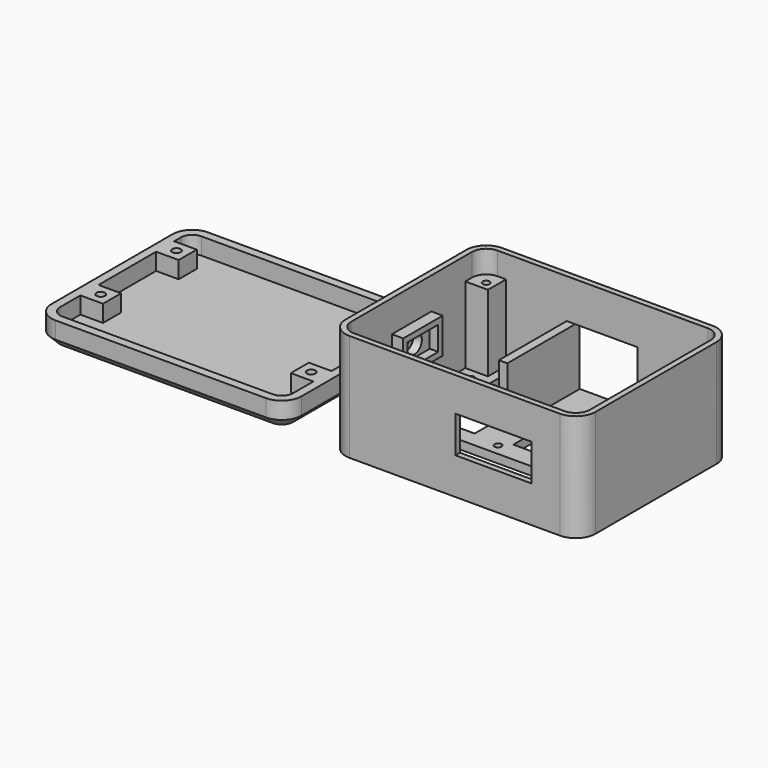
from build123d import *

# Parameters (mm, degrees)
F0_R      = 1.5
F1_DEPTH  = 3
F2_DEPTH  = 38
F0_R_2    = 1.25
F3_DEPTH  = 30
F4_W      = 21
F4_H      = 17
F5_DEPTH  = 7
F7_DEPTH  = 3
F8_W      = 4
F8_H      = 9
F9_DEPTH  = 25
F10_SIZE  = 1.5
F12_W     = 21
F12_H     = 21
F13_DEPTH = 25
F14_DEPTH = 25
F15_R     = 1.5
F15_R_2   = 1.25
F16_DEPTH = 3
F15_W     = 8
F15_H     = 8
F17_DEPTH = 9
F18_SIZE  = 3
F19_DEPTH = 25
F8_W_2    = 17.5
F8_H_2    = 12.5
F8_W_3    = 13.5
F8_H_3    = 8.5
F20_DEPTH = 4
F8_R      = 3.25
F21_DEPTH = 25
F23_DEPTH = 8
F24_DEPTH = 1
F25_DEPTH = 1
F26_DEPTH = 1
F27_DEPTH = 1
F28_DEPTH = 1
F29_W     = 3
F29_H     = 30
F30_DEPTH = 21
F31_DEPTH = 1
F29_W_2   = 15.5
F29_H_2   = 34
F32_DEPTH = 25
F33_DEPTH = 25
F11_W     = 39
F11_H     = 21
F34_DEPTH = 25
F36_DEPTH = 25


# Not quite as in the source:
# - a feature names something its author has since deleted; it is built from what else it names


with BuildPart() as f1:
    # F0 (on Top) → F1 (new body)
    with BuildSketch(Plane.XY):
        Polygon((-34.25, -30.75), (34.25, -30.75), (34.25, -23.75), (41.25, -23.75), (41.25, 23.75), (34.25, 23.75), (34.25, 30.75), (-34.25, 30.75), (-34.25, 23.75), (-41.25, 23.75), (-41.25, -23.75), (-34.25, -23.75), align=None)
        with Locations((-37.25, -13.75)):
            Circle(F0_R, mode=Mode.SUBTRACT)
        with Locations((37.25, -13.75)):
            Circle(F0_R, mode=Mode.SUBTRACT)
        with Locations((-37.25, 19.75)):
            Circle(F0_R, mode=Mode.SUBTRACT)
        with Locations((30.25, 26.75)):
            Circle(F0_R, mode=Mode.SUBTRACT)
    extrude(amount=F1_DEPTH)

    # F0 (on Top) → F2 (join)
    with BuildSketch(Plane.XY):
        with BuildLine():
            Line((44.25, -26.75), (44.25, 26.75))
            ThreePointArc((44.25, 26.75), (42.1997474683, 31.6997474683), (37.25, 33.75))
            Line((37.25, 33.75), (-37.25, 33.75))
            ThreePointArc((-37.25, 33.75), (-42.1997474683, 31.6997474683), (-44.25, 26.75))
            Line((-44.25, 26.75), (-44.25, -26.75))
            ThreePointArc((-44.25, -26.75), (-42.1997474683, -31.6997474683), (-37.25, -33.75))
            Line((-37.25, -33.75), (37.25, -33.75))
            ThreePointArc((37.25, -33.75), (42.1997474683, -31.6997474683), (44.25, -26.75))
        make_face()
        with BuildLine():
            ThreePointArc((41.25, -26.75), (40.0784271247, -29.5784271247), (37.25, -30.75))
            Line((37.25, -30.75), (34.25, -30.75))
            Line((34.25, -30.75), (-34.25, -30.75))
            Line((-34.25, -30.75), (-37.25, -30.75))
            ThreePointArc((-37.25, -30.75), (-40.0784271247, -29.5784271247), (-41.25, -26.75))
            Line((-41.25, -26.75), (-41.25, -23.75))
            Line((-41.25, -23.75), (-41.25, 23.75))
            Line((-41.25, 23.75), (-41.25, 26.75))
            ThreePointArc((-41.25, 26.75), (-40.0784271247, 29.5784271247), (-37.25, 30.75))
            Line((-37.25, 30.75), (-34.25, 30.75))
            Line((-34.25, 30.75), (34.25, 30.75))
            Line((34.25, 30.75), (37.25, 30.75))
            ThreePointArc((37.25, 30.75), (40.0784271247, 29.5784271247), (41.25, 26.75))
            Line((41.25, 26.75), (41.25, 23.75))
            Line((41.25, 23.75), (41.25, -23.75))
            Line((41.25, -23.75), (41.25, -26.75))
        make_face(mode=Mode.SUBTRACT)
    extrude(amount=F2_DEPTH)

    # F0 (on Top) → F3 (join)
    with BuildSketch(Plane.XY):
        with BuildLine():
            Line((-41.25, 26.75), (-41.25, 23.75))
            Line((-41.25, 23.75), (-34.25, 23.75))
            Line((-34.25, 23.75), (-34.25, 30.75))
            Line((-34.25, 30.75), (-37.25, 30.75))
            ThreePointArc((-37.25, 30.75), (-40.0784271247, 29.5784271247), (-41.25, 26.75))
        make_face()
        with Locations((-37.25, 26.75)):
            Circle(F0_R_2, mode=Mode.SUBTRACT)
        with BuildLine():
            Line((-37.25, -30.75), (-34.25, -30.75))
            Line((-34.25, -30.75), (-34.25, -23.75))
            Line((-34.25, -23.75), (-41.25, -23.75))
            Line((-41.25, -23.75), (-41.25, -26.75))
            ThreePointArc((-41.25, -26.75), (-40.0784271247, -29.5784271247), (-37.25, -30.75))
        make_face()
        with Locations((-37.25, -26.75)):
            Circle(F0_R_2, mode=Mode.SUBTRACT)
        with BuildLine():
            Line((34.25, 23.75), (41.25, 23.75))
            Line((41.25, 23.75), (41.25, 26.75))
            ThreePointArc((41.25, 26.75), (40.0784271247, 29.5784271247), (37.25, 30.75))
            Line((37.25, 30.75), (34.25, 30.75))
            Line((34.25, 30.75), (34.25, 23.75))
        make_face()
        with Locations((37.25, 26.75)):
            Circle(F0_R_2, mode=Mode.SUBTRACT)
        with BuildLine():
            Line((34.25, -30.75), (37.25, -30.75))
            ThreePointArc((37.25, -30.75), (40.0784271247, -29.5784271247), (41.25, -26.75))
            Line((41.25, -26.75), (41.25, -23.75))
            Line((41.25, -23.75), (34.25, -23.75))
            Line((34.25, -23.75), (34.25, -30.75))
        make_face()
        with Locations((37.25, -26.75)):
            Circle(F0_R_2, mode=Mode.SUBTRACT)
    extrude(amount=F3_DEPTH)

    # F4 (on face) → F5 (join)
    with BuildSketch(Plane(origin=(0, -30.75, 0), x_dir=(-1, 0, 0), z_dir=(0, 1, 0))):
        Polygon((10.25, 3), (13.25, 3), (13.25, 20), (34.25, 20), (34.25, 23), (10.25, 23), align=None)
        with Locations((23.75, 11.5)):
            Rectangle(F4_W, F4_H)
    extrude(amount=F5_DEPTH)

    # F6 (on face) → F7 (join)
    with BuildSketch(Plane(origin=(0, -23.75, 0), x_dir=(-1, 0, 0), z_dir=(0, 1, 0))):
        Polygon((41.25, 23), (34.25, 23), (10.25, 23), (10.25, 3), (13.25, 3), (13.25, 20), (41.25, 20), align=None)
    extrude(amount=F7_DEPTH)

    # F8 (on face) → F9 (cut)
    with BuildSketch(Plane.YZ.offset(-41.25)):
        with Locations((-20.75, 11.5)):
            Rectangle(F8_W, F8_H)
    extrude(amount=-F9_DEPTH, mode=Mode.SUBTRACT)

    # F10
    f10_edges = [f1.edges().sort_by_distance(p)[0] for p in [
        (-44.25, -18.75, 11.5),
        (-44.25, -20.75, 7),
        (-44.25, -22.75, 11.5),
        (-44.25, -20.75, 16),
    ]]
    chamfer(f10_edges, length=F10_SIZE)

    # F12 (on face) → F13 (cut)
    with BuildSketch(Plane.XZ.offset(-30.75)):
        with Locations((1.75, 13.5)):
            Rectangle(F12_W, F12_H)
    extrude(amount=-F13_DEPTH, mode=Mode.SUBTRACT)

    # F4 (on face) → F14 (cut)
    with BuildSketch(Plane(origin=(0, -30.75, 0), x_dir=(-1, 0, 0), z_dir=(0, 1, 0))):
        Polygon((-0.25, 26), (-3.25, 26), (-27.25, 26), (-27.25, 16), (-27.25, 13), (-0.25, 13), align=None)
    extrude(amount=-F14_DEPTH, mode=Mode.SUBTRACT)

    # F11 (on face) → F19 (cut)
    with BuildSketch(Plane.XY.offset(3)):
        with BuildLine():
            Line((38.75, 20.25), (40, 20.25))
            ThreePointArc((40, 20.25), (38.75, 21.5), (37.5, 20.25))
            Line((37.5, 20.25), (38.75, 20.25))
        make_face()
        with BuildLine():
            Line((38.75, 20.25), (37.5, 20.25))
            ThreePointArc((37.5, 20.25), (37.8661165235, 19.3661165235), (38.75, 19))
            Line((38.75, 19), (38.75, 20.25))
        make_face()
        with BuildLine():
            ThreePointArc((38.75, 19), (39.6338834765, 19.3661165235), (40, 20.25))
            Line((40, 20.25), (38.75, 20.25))
            Line((38.75, 20.25), (38.75, 19))
        make_face()
    extrude(amount=-F19_DEPTH, mode=Mode.SUBTRACT)

    # F8 (on face) → F20 (join)
    with BuildSketch(Plane.YZ.offset(-41.25)):
        with Locations((0, 20.5)):
            Rectangle(F8_W_2, F8_H_2)
        with Locations((0, 20.5)):
            Rectangle(F8_W_3, F8_H_3, mode=Mode.SUBTRACT)
    extrude(amount=F20_DEPTH)

    # F8 (on face) → F21 (cut)
    with BuildSketch(Plane.YZ.offset(-41.25)):
        with Locations((0, 20.5)):
            Circle(F8_R)
    extrude(amount=-F21_DEPTH, mode=Mode.SUBTRACT)

    # F22 (on face) → F23 (cut)
    with BuildSketch(Plane.XY.offset(38)):
        with BuildLine():
            Line((-42.25, 26.75), (-42.25, -26.75))
            ThreePointArc((-42.25, -26.75), (-40.7855339059, -30.2855339059), (-37.25, -31.75))
            Line((-37.25, -31.75), (37.25, -31.75))
            ThreePointArc((37.25, -31.75), (40.7855339059, -30.2855339059), (42.25, -26.75))
            Line((42.25, -26.75), (42.25, 26.75))
            ThreePointArc((42.25, 26.75), (40.7855339059, 30.2855339059), (37.25, 31.75))
            Line((37.25, 31.75), (-37.25, 31.75))
            ThreePointArc((-37.25, 31.75), (-40.7855339059, 30.2855339059), (-42.25, 26.75))
        make_face()
        with BuildLine():
            Line((41.25, 26.75), (41.25, -26.75))
            ThreePointArc((41.25, -26.75), (40.0784271247, -29.5784271247), (37.25, -30.75))
            Line((37.25, -30.75), (-37.25, -30.75))
            ThreePointArc((-37.25, -30.75), (-40.0784271247, -29.5784271247), (-41.25, -26.75))
            Line((-41.25, -26.75), (-41.25, 26.75))
            ThreePointArc((-41.25, 26.75), (-40.0784271247, 29.5784271247), (-37.25, 30.75))
            Line((-37.25, 30.75), (37.25, 30.75))
            ThreePointArc((37.25, 30.75), (40.0784271247, 29.5784271247), (41.25, 26.75))
        make_face(mode=Mode.SUBTRACT)
    extrude(amount=-F23_DEPTH, mode=Mode.SUBTRACT)

    # F24 (cut): a face of the model
    f24_faces = [f1.faces().sort_by_distance(p)[0] for p in [
        (-41.25, -22.25, 23.5463744137),
    ]]
    extrude(f24_faces, amount=-F24_DEPTH, mode=Mode.SUBTRACT)

    # F25 (cut): a face of the model
    f25_faces = [f1.faces().sort_by_distance(p)[0] for p in [
        (-21.5, 30.75, 3.7362913825),
    ]]
    extrude(f25_faces, amount=-F25_DEPTH, mode=Mode.SUBTRACT)

    # F26 (cut): a face of the model
    f26_faces = [f1.faces().sort_by_distance(p)[0] for p in [
        (41.25, 0, 16.5),
    ]]
    extrude(f26_faces, amount=-F26_DEPTH, mode=Mode.SUBTRACT)

    # F27 (cut): a face of the model
    f27_faces = [f1.faces().sort_by_distance(p)[0] for p in [
        (12, -30.75, 3.7362913825),
    ]]
    extrude(f27_faces, amount=-F27_DEPTH, mode=Mode.SUBTRACT)

    # F28 (cut): a face of the model
    f28_faces = [f1.faces().sort_by_distance(p)[0] for p in [
        (-37.25, 0, 26.5349418683),
    ]]
    extrude(f28_faces, amount=-F28_DEPTH, mode=Mode.SUBTRACT)

    # F29 (on face) → F30 (join)
    with BuildSketch(Plane.XY.offset(3)):
        with Locations((-11.25, 16.75)):
            Rectangle(F29_W, F29_H)
    extrude(amount=F30_DEPTH)

    # F31 (cut): a face of the model
    f31_faces = [f1.faces().sort_by_distance(p)[0] for p in [
        (-8.75, 32.75, 13.5),
    ]]
    extrude(f31_faces, amount=-F31_DEPTH, mode=Mode.SUBTRACT)

    # F29 (on face) → F32 (cut)
    with BuildSketch(Plane.XY.offset(3)):
        with Locations((-23.5, 11.75)):
            Rectangle(F29_W_2, F29_H_2)
    extrude(amount=-F32_DEPTH, mode=Mode.SUBTRACT)

    # F11 (on face) → F33 (cut)
    with BuildSketch(Plane.XY.offset(3)):
        with BuildLine():
            ThreePointArc((-5, -6.75), (-5.3661165235, -5.8661165235), (-6.25, -5.5))
            Line((-6.25, -5.5), (-6.25, -6.75))
            Line((-6.25, -6.75), (-5, -6.75))
        make_face()
        with BuildLine():
            ThreePointArc((-6.25, -5.5), (-7.5, -6.75), (-6.25, -8))
            Line((-6.25, -8), (-6.25, -6.75))
            Line((-6.25, -6.75), (-6.25, -5.5))
        make_face()
        with BuildLine():
            Line((-6.25, -6.75), (-6.25, -8))
            ThreePointArc((-6.25, -8), (-5.3661165235, -7.6338834765), (-5, -6.75))
            Line((-5, -6.75), (-6.25, -6.75))
        make_face()
    extrude(amount=-F33_DEPTH, mode=Mode.SUBTRACT)

    # F11 (on face) → F34 (cut)
    with BuildSketch(Plane.XY.offset(3)):
        with Locations((16.25, 6.75)):
            Rectangle(F11_W, F11_H)
    extrude(amount=-F34_DEPTH, mode=Mode.SUBTRACT)

    # F35 (on face) → F36 (cut)
    with BuildSketch(Plane.XY.offset(3)):
        Polygon((-31.25, -10.75), (-31.25, -20.75), (-13.25, -20.75), (-10.25, -20.75), (31.75, -20.75), (31.75, -10.75), align=None)
    extrude(amount=-F36_DEPTH, mode=Mode.SUBTRACT)


with BuildPart() as f16:
    # F15 (on Top) → F16 (new body)
    with BuildSketch(Plane.XY):
        Polygon((-138.3466287255, -30.75), (-69.8466287255, -30.75), (-69.8466287255, -23.75), (-62.8466287255, -23.75), (-62.8466287255, -17.75), (-70.8466287255, -17.75), (-70.8466287255, -9.75), (-62.8466287255, -9.75), (-62.8466287255, -3.75), (-62.8466287255, 15.75), (-62.8466287255, 23.75), (-69.8466287255, 23.75), (-69.8466287255, 22.75), (-77.8466287255, 22.75), (-77.8466287255, 30.75), (-138.3466287255, 30.75), (-138.3466287255, 23.75), (-137.3466287255, 23.75), (-137.3466287255, 15.75), (-145.3466287255, 15.75), (-145.3466287255, -9.75), (-137.3466287255, -9.75), (-137.3466287255, -17.75), (-145.3466287255, -17.75), (-145.3466287255, -23.75), (-138.3466287255, -23.75), align=None)
        Polygon((-69.8466287255, 22.75), (-69.8466287255, 23.75), (-69.8466287255, 30.75), (-77.8466287255, 30.75), (-77.8466287255, 22.75), align=None)
        with Locations((-73.8466287255, 26.75)):
            Circle(F15_R, mode=Mode.SUBTRACT)
        with BuildLine():
            Line((-69.8466287255, 23.75), (-62.8466287255, 23.75))
            Line((-62.8466287255, 23.75), (-62.8466287255, 26.75))
            ThreePointArc((-62.8466287255, 26.75), (-64.0182016008, 29.5784271247), (-66.8466287255, 30.75))
            Line((-66.8466287255, 30.75), (-69.8466287255, 30.75))
            Line((-69.8466287255, 30.75), (-69.8466287255, 23.75))
        make_face()
        with Locations((-66.8466287255, 26.75)):
            Circle(F15_R_2, mode=Mode.SUBTRACT)
        with BuildLine():
            Line((-69.8466287255, -30.75), (-66.8466287255, -30.75))
            ThreePointArc((-66.8466287255, -30.75), (-64.0182016008, -29.5784271247), (-62.8466287255, -26.75))
            Line((-62.8466287255, -26.75), (-62.8466287255, -23.75))
            Line((-62.8466287255, -23.75), (-69.8466287255, -23.75))
            Line((-69.8466287255, -23.75), (-69.8466287255, -30.75))
        make_face()
        with Locations((-66.8466287255, -26.75)):
            Circle(F15_R_2, mode=Mode.SUBTRACT)
        with BuildLine():
            Line((-141.3466287255, -30.75), (-138.3466287255, -30.75))
            Line((-138.3466287255, -30.75), (-138.3466287255, -23.75))
            Line((-138.3466287255, -23.75), (-145.3466287255, -23.75))
            Line((-145.3466287255, -23.75), (-145.3466287255, -26.75))
            ThreePointArc((-145.3466287255, -26.75), (-144.1750558503, -29.5784271247), (-141.3466287255, -30.75))
        make_face()
        with Locations((-141.3466287255, -26.75)):
            Circle(F15_R_2, mode=Mode.SUBTRACT)
        with BuildLine():
            Line((-145.3466287255, 26.75), (-145.3466287255, 23.75))
            Line((-145.3466287255, 23.75), (-138.3466287255, 23.75))
            Line((-138.3466287255, 23.75), (-138.3466287255, 30.75))
            Line((-138.3466287255, 30.75), (-141.3466287255, 30.75))
            ThreePointArc((-141.3466287255, 30.75), (-144.1750558503, 29.5784271247), (-145.3466287255, 26.75))
        make_face()
        with Locations((-141.3466287255, 26.75)):
            Circle(F15_R_2, mode=Mode.SUBTRACT)
        with Locations((-66.8466287255, 26.75)):
            Circle(F15_R_2)
        with Locations((-66.8466287255, -26.75)):
            Circle(F15_R_2)
        with Locations((-141.3466287255, -26.75)):
            Circle(F15_R_2)
        with Locations((-141.3466287255, 26.75)):
            Circle(F15_R_2)
    extrude(amount=F16_DEPTH)

    # F15 (on Top) → F17 (join)
    with BuildSketch(Plane.XY):
        with BuildLine():
            Line((-59.8466287255, -26.75), (-59.8466287255, 26.75))
            ThreePointArc((-59.8466287255, 26.75), (-61.8968812572, 31.6997474683), (-66.8466287255, 33.75))
            Line((-66.8466287255, 33.75), (-141.3466287255, 33.75))
            ThreePointArc((-141.3466287255, 33.75), (-146.2963761938, 31.6997474683), (-148.3466287255, 26.75))
            Line((-148.3466287255, 26.75), (-148.3466287255, -26.75))
            ThreePointArc((-148.3466287255, -26.75), (-146.2963761938, -31.6997474683), (-141.3466287255, -33.75))
            Line((-141.3466287255, -33.75), (-66.8466287255, -33.75))
            ThreePointArc((-66.8466287255, -33.75), (-61.8968812572, -31.6997474683), (-59.8466287255, -26.75))
        make_face()
        with BuildLine():
            ThreePointArc((-62.8466287255, -26.75), (-64.0182016008, -29.5784271247), (-66.8466287255, -30.75))
            Line((-66.8466287255, -30.75), (-69.8466287255, -30.75))
            Line((-69.8466287255, -30.75), (-138.3466287255, -30.75))
            Line((-138.3466287255, -30.75), (-141.3466287255, -30.75))
            ThreePointArc((-141.3466287255, -30.75), (-144.1750558503, -29.5784271247), (-145.3466287255, -26.75))
            Line((-145.3466287255, -26.75), (-145.3466287255, -23.75))
            Line((-145.3466287255, -23.75), (-145.3466287255, -17.75))
            Line((-145.3466287255, -17.75), (-145.3466287255, -9.75))
            Line((-145.3466287255, -9.75), (-145.3466287255, 15.75))
            Line((-145.3466287255, 15.75), (-145.3466287255, 23.75))
            Line((-145.3466287255, 23.75), (-145.3466287255, 26.75))
            ThreePointArc((-145.3466287255, 26.75), (-144.1750558503, 29.5784271247), (-141.3466287255, 30.75))
            Line((-141.3466287255, 30.75), (-138.3466287255, 30.75))
            Line((-138.3466287255, 30.75), (-77.8466287255, 30.75))
            Line((-77.8466287255, 30.75), (-69.8466287255, 30.75))
            Line((-69.8466287255, 30.75), (-66.8466287255, 30.75))
            ThreePointArc((-66.8466287255, 30.75), (-64.0182016008, 29.5784271247), (-62.8466287255, 26.75))
            Line((-62.8466287255, 26.75), (-62.8466287255, 23.75))
            Line((-62.8466287255, 23.75), (-62.8466287255, 15.75))
            Line((-62.8466287255, 15.75), (-62.8466287255, -3.75))
            Line((-62.8466287255, -3.75), (-62.8466287255, -9.75))
            Line((-62.8466287255, -9.75), (-62.8466287255, -17.75))
            Line((-62.8466287255, -17.75), (-62.8466287255, -23.75))
            Line((-62.8466287255, -23.75), (-62.8466287255, -26.75))
        make_face(mode=Mode.SUBTRACT)
        with Locations((-141.3466287255, -13.75)):
            Rectangle(F15_W, F15_H)
        with Locations((-141.3466287255, -13.75)):
            Circle(F15_R, mode=Mode.SUBTRACT)
        Polygon((-145.3466287255, 23.75), (-145.3466287255, 15.75), (-137.3466287255, 15.75), (-137.3466287255, 23.75), (-138.3466287255, 23.75), align=None)
        with Locations((-141.3466287255, 19.75)):
            Circle(F15_R, mode=Mode.SUBTRACT)
        with Locations((-66.8466287255, -13.75)):
            Rectangle(F15_W, F15_H)
        with Locations((-66.8466287255, -13.75)):
            Circle(F15_R, mode=Mode.SUBTRACT)
        Polygon((-69.8466287255, 22.75), (-69.8466287255, 23.75), (-69.8466287255, 30.75), (-77.8466287255, 30.75), (-77.8466287255, 22.75), align=None)
        with Locations((-73.8466287255, 26.75)):
            Circle(F15_R, mode=Mode.SUBTRACT)
    extrude(amount=F17_DEPTH)

    # F18
    f18_edges = [f16.edges().sort_by_distance(p)[0] for p in [
        (-104.096629, -33.75, 0),
        (-61.896881, -31.699747, 0),
        (-59.846629, 0, 0),
        (-61.896881, 31.699747, 0),
        (-104.096629, 33.75, 0),
        (-146.296376, 31.699747, 0),
        (-148.346629, 0, 0),
        (-146.296376, -31.699747, 0),
    ]]
    chamfer(f18_edges, length=F18_SIZE)


solid = Compound([f1.part, f16.part])
